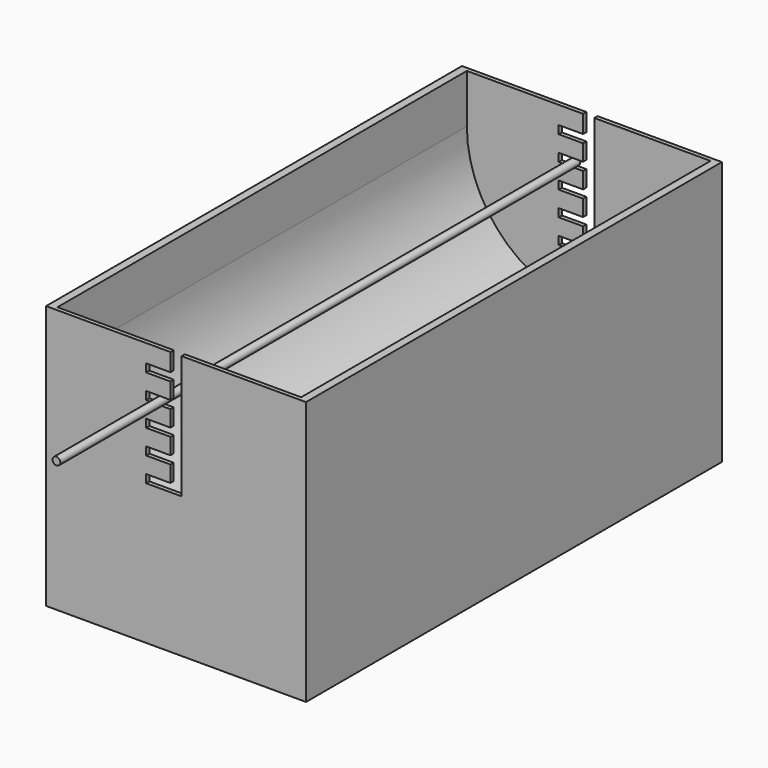
from build123d import *

# Parameters (mm, degrees)
F0_W      = 203.2
F0_H      = 406.4
F0_W_2    = 196.85
F0_H_2    = 400.05
F1_DEPTH  = 203.2
F2_W      = 203.2
F2_H      = 3.175
F3_DEPTH  = 406.4
F5_DEPTH  = 406.401
F7_DEPTH  = 400.05
F8_R      = 3.048
F9_DEPTH  = 508
F10_ANGLE = 180


# Not quite as in the source:
# - a feature names something its author has since deleted; it is built from what else it names


with BuildPart() as f1:
    # F0 (on Top) → F1 (new body)
    with BuildSketch(Plane.XY):
        Rectangle(F0_W, F0_H)
        Rectangle(F0_W_2, F0_H_2, mode=Mode.SUBTRACT)
    extrude(amount=F1_DEPTH)

    # F2 (on face) → F3 (join)
    with BuildSketch(Plane.XZ.offset(203.2)):
        with Locations((0, 204.7875)):
            Rectangle(F2_W, F2_H)
    extrude(amount=-F3_DEPTH)

    # F4 (on face) → F5 (cut, through all)
    with BuildSketch(Plane(origin=(0, 203.2, 0), x_dir=(-1, 0, 0), z_dir=(0, 1, 0))):
        Polygon((-4.3847840279, 0), (4.3847840279, 0), (4.3847840279, 96.4816804707), (-4.3847840279, 96.4816804707), (-23.4347840279, 96.4816804707), (-23.4347840279, 90.1316804707), (-4.3847840279, 90.1316804707), (-4.3847840279, 77.4316804707), (-23.4347840279, 77.4316804707), (-23.4347840279, 71.0816804707), (-4.3847840279, 71.0816804707), (-4.3847840279, 58.3816804707), (-23.4347840279, 58.3816804707), (-23.4347840279, 52.0316804707), (-4.3847840279, 52.0316804707), (-4.3847840279, 39.3316804707), (-23.4347840279, 39.3316804707), (-23.4347840279, 32.9816804707), (-4.3847840279, 32.9816804707), (-4.3847840279, 20.2816804707), (-23.4347840279, 20.2816804707), (-23.4347840279, 13.9316804707), (-4.3847840279, 13.9316804707), align=None)
    extrude(amount=-F5_DEPTH, mode=Mode.SUBTRACT)

    # F6 (on face) → F7 (join, through all)
    with BuildSketch(Plane.XZ.offset(-200.025)):
        with BuildLine():
            Line((95.25, 0), (98.425, 0))
            Line((98.425, 0), (98.425, 38.1))
            ThreePointArc((98.425, 38.1), (0, 136.525), (-98.425, 38.1))
            Line((-98.425, 38.1), (-98.425, 0))
            Line((-98.425, 0), (-95.25, 0))
            Line((-95.25, 0), (-95.25, 38.1))
            ThreePointArc((-95.25, 38.1), (0, 133.35), (95.25, 38.1))
            Line((95.25, 38.1), (95.25, 0))
        make_face()
    extrude(amount=F7_DEPTH)

    # F8 (on face) → F9 (join)
    with BuildSketch(Plane(origin=(0, 203.2, 0), x_dir=(-1, 0, 0), z_dir=(0, 1, 0))):
        with Locations((-12.1751278639, 36.2836804707)):
            Circle(F8_R)
    extrude(amount=-F9_DEPTH)


with BuildPart() as f1_1:
    # F10: moved
    add(f1.part.rotate(Axis((12.1751278639, 203.2, 36.2836804707), (0, 1, 0)), F10_ANGLE))


solid = f1_1.part
